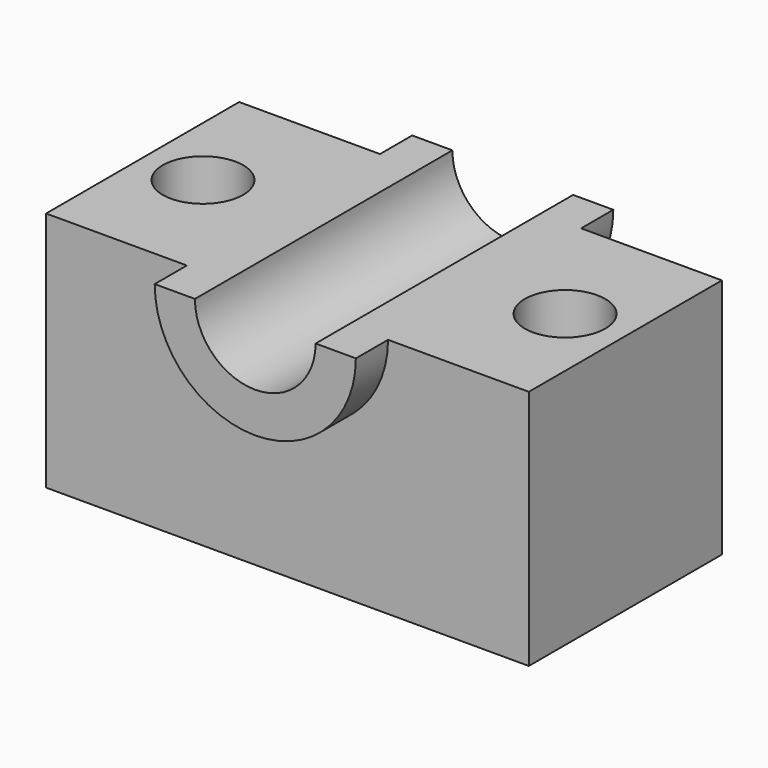
from build123d import *

# Parameters (mm, degrees)
F0_W     = 304.8
F0_H     = 152.4
F0_R     = 25.4
F1_DEPTH = 152.4
F3_DEPTH = 101.6
F4_DEPTH = 177.801


with BuildPart() as f1:
    # F0 (on Top) → F1 (new body)
    with BuildSketch(Plane.XY):
        Rectangle(F0_W, F0_H)
        with Locations((-114.3, 0)):
            Circle(F0_R, mode=Mode.SUBTRACT)
        with Locations((114.3, 0)):
            Circle(F0_R, mode=Mode.SUBTRACT)
    extrude(amount=F1_DEPTH)

    # F2 (on Front) → F3 (join, symmetric)
    with BuildSketch(Plane.XZ):
        with BuildLine():
            Line((63.5, 152.4), (38.1, 152.4))
            ThreePointArc((38.1, 152.4), (0, 114.3), (-38.1, 152.4))
            Line((-38.1, 152.4), (-63.5, 152.4))
            ThreePointArc((-63.5, 152.4), (0, 88.9), (63.5, 152.4))
        make_face()
    extrude(amount=F3_DEPTH, both=True)

    # F4 (cut, through all): a face of the model
    f4_faces = [f1.faces().sort_by_distance(p)[0] for p in [
        (0, -76.2, 136.2298577819),
    ]]
    extrude(f4_faces, amount=-F4_DEPTH, mode=Mode.SUBTRACT)


solid = f1.part
